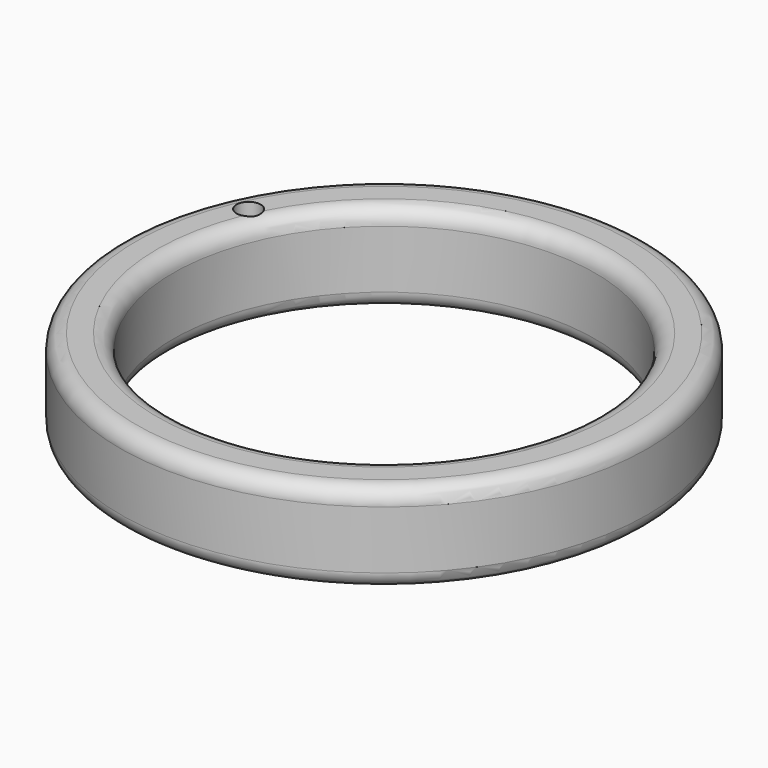
from build123d import *

# Parameters (mm, degrees)
F0_R     = 50
F0_R_2   = 2.2916267838
F0_R_3   = 40
F1_DEPTH = 17


# Not quite as in the source:
# - a fillet or chamfer that OpenCascade refuses, or shapes differently, is made with other operations: its cross-section is extruded or revolved along the edge and cut away or added


with BuildPart() as f1:
    # F0 (on Top) → F1 (new body)
    with BuildSketch(Plane.XY):
        Circle(F0_R)
        with Locations((-40.46940431, 18.5024235398)):
            Circle(F0_R_2, mode=Mode.SUBTRACT)
        Circle(F0_R_3, mode=Mode.SUBTRACT)
    extrude(amount=F1_DEPTH)

    # F2: fillet of radius 3 on 5 edges, made by hand

    # F2_s1 → F2_t2 (revolve, cut)
    with BuildSketch(Plane.XZ):
        with BuildLine():
            ThreePointArc((50, 3), (49.1213203436, 0.8786796564), (47, 0))
            Line((47, 0), (50, 0))
            Line((50, 0), (50, 3))
        make_face()
    revolve(axis=Axis((0, 0, 0), (0, 0, 1)), mode=Mode.SUBTRACT)

    # F2_s3 → F2_t4 (revolve, cut)
    with BuildSketch(Plane.XZ):
        with BuildLine():
            ThreePointArc((50, 14), (49.1213203436, 16.1213203436), (47, 17))
            Line((47, 17), (50, 17))
            Line((50, 17), (50, 14))
        make_face()
    revolve(axis=Axis((0, 0, 17), (0, 0, 1)), mode=Mode.SUBTRACT)

    # F2_s5 → F2_t6 (revolve, cut)
    with BuildSketch(Plane.XZ):
        with BuildLine():
            ThreePointArc((40, 14), (40.8786796564, 16.1213203436), (43, 17))
            Line((43, 17), (40, 17))
            Line((40, 17), (40, 14))
        make_face()
    revolve(axis=Axis((0, 0, 17), (0, 0, 1)), mode=Mode.SUBTRACT)

    # F2_s7 → F2_t8 (revolve, cut)
    with BuildSketch(Plane.XZ):
        with BuildLine():
            ThreePointArc((40, 3), (40.8786796564, 0.8786796564), (43, 0))
            Line((43, 0), (40, 0))
            Line((40, 0), (40, 3))
        make_face()
    revolve(axis=Axis((0, 0, 0), (0, 0, 1)), mode=Mode.SUBTRACT)


solid = f1.part
